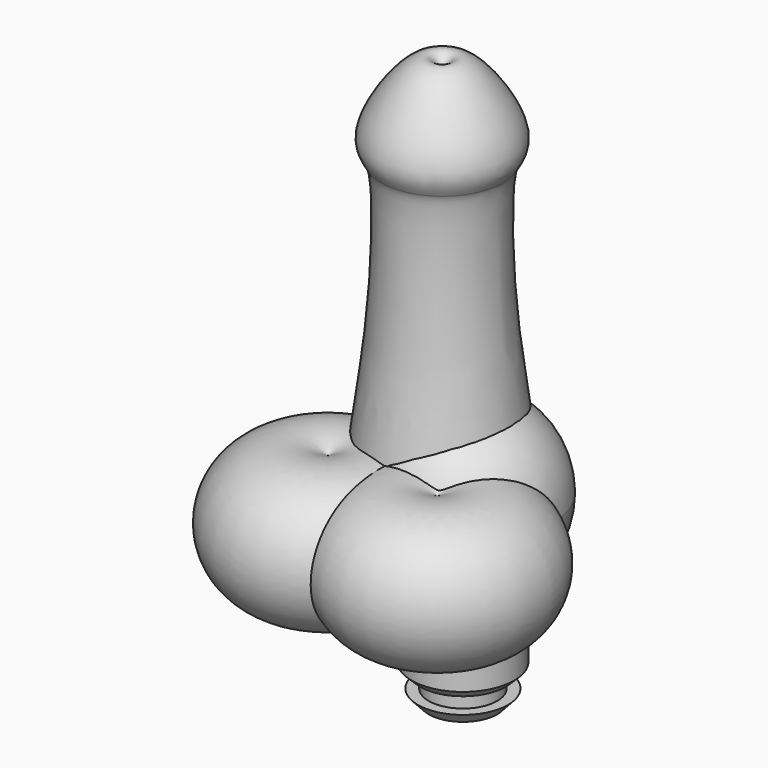
from build123d import *

# Parameters (mm, degrees)
F2_R     = 15
F3_R     = 5.5319781754
F4_DEPTH = 47.3


with BuildPart() as f1:
    # F0 (on Front) → F1 (revolve)
    with BuildSketch(Plane.XZ):
        with BuildLine():
            ThreePointArc((11.6922361776, -16.2262630685), (17.8023133827, -9.1146935343), (20, 0))
            ThreePointArc((20, 0), (14.1421356237, 14.1421356237), (0, 20))
            Line((0, 20), (0, 12.6605455616))
            Line((0, 12.6605455616), (11.6922361776, 12.6605455616))
            Line((11.6922361776, 12.6605455616), (11.6922361776, -16.2262630685))
        make_face()
        with BuildLine():
            ThreePointArc((0, -20), (6.1430749072, -19.0331981202), (11.6922361776, -16.2262630685))
            Line((11.6922361776, -16.2262630685), (11.6922361776, 12.6605455616))
            Line((11.6922361776, 12.6605455616), (0, 12.6605455616))
            Line((0, 12.6605455616), (0, -20))
        make_face()
        with BuildLine():
            Line((11.6922361776, -34.058239311), (11.6922361776, -16.2262630685))
            ThreePointArc((11.6922361776, -16.2262630685), (6.1430749072, -19.0331981202), (0, -20))
            Line((0, -20), (0, -35.9514871388))
            Line((0, -35.9514871388), (7.8149475157, -35.9514871388))
            Line((7.8149475157, -35.9514871388), (9.7362715751, -35.9514871388))
            Line((9.7362715751, -35.9514871388), (11.6922361776, -34.058239311))
        make_face()
        Polygon((7.8149475157, -35.9514871388), (0, -35.9514871388), (0, -42.1006083488), (7.8149475157, -42.1006083488), (10.26965864, -39.4199751318), (7.8149475157, -39.4199751318), align=None)
    revolve(axis=Axis((0, 0, -7.9757435694), (0, 0, -1)))

    # F2
    f2_edges = [f1.edges().sort_by_distance(p)[0] for p in [
        (-11.692236, 0, -16.226263),
    ]]
    fillet(f2_edges, radius=F2_R)

    # F3 (on face) → F4 (cut)
    with BuildSketch(Plane(origin=(0, 0, -42.1006083488), x_dir=(1, 0, 0), z_dir=(0, 0, -1))):
        Circle(F3_R)
    extrude(amount=-F4_DEPTH, mode=Mode.SUBTRACT)


with BuildPart() as f6:
    # F5 (on Front) → F6 (revolve)
    with BuildSketch(Plane.XZ):
        with BuildLine():
            Line((-4.7232788056, 65.1360228658), (-4.7232788056, -18.2994715869))
            Line((-4.7232788056, -18.2994715869), (12.0858419687, -18.2994715869))
            add(Edge.make_bspline(
                [(12.0858419687, -18.2994715869), (12.9072001435, -16.5504610424), (15.8298986021, -10.3268297703), (7.1919181413, 32.3844006338), (7.6965663946, 63.4385033004), (9.138613008, 65.1360228658)],
                knots=[0, 0, 0, 0, 0.1680965129, 0.5981500327, 0.9442662694, 0.9442662694, 0.9442662694, 0.9442662694], degree=3))
            add(Edge.make_bspline(
                [(9.138613008, 65.1360228658), (10.2272078713, 66.9279335369), (13.0840514311, 71.6305172372), (-1.2602489922, 91.110867704), (-4.608384321, 82.8719045533), (-4.7232788056, 82.8164368868)],
                knots=[0, 0, 0, 0, 0.2817011042, 0.7392796094, 0.9609287933, 0.9609287933, 0.9609287933, 0.9609287933], degree=3))
            Line((-4.7232788056, 82.8164368868), (-4.7232788056, 65.1360228658))
        make_face()
    revolve(axis=Axis((-4.7232788056, 0, 73.9762298763), (0, 0, -1)))


with BuildPart() as f12:
    # F11 (on offset) → F12 (revolve)
    with BuildSketch(Plane.XZ.offset(17)):
        with BuildLine():
            Line((7.78110791, -3.4937250894), (7.78110791, -18.2994715869))
            Line((7.78110791, -18.2994715869), (12.0858419687, -18.2994715869))
            Line((12.0858419687, -18.2994715869), (22.0654299709, -18.2994715869))
            Line((22.0654299709, -18.2994715869), (24.2403661832, -18.2994715869))
            ThreePointArc((24.2403661832, -18.2994715869), (29.5091951266, 3.4286156297), (7.78110791, 8.697444573))
            Line((7.78110791, 8.697444573), (7.78110791, -3.4937250894))
        make_face()
    revolve(axis=Axis((7.78110791, -17, 2.6018597418), (0, 0, 1)))

    # F13: F12 across plane


with BuildPart() as f12_1:
    add(f12.part)
    add(f12.part.mirror(Plane.YZ.offset(-4.7232788056)))


solid = Compound([f1.part, f6.part, f12_1.part])
